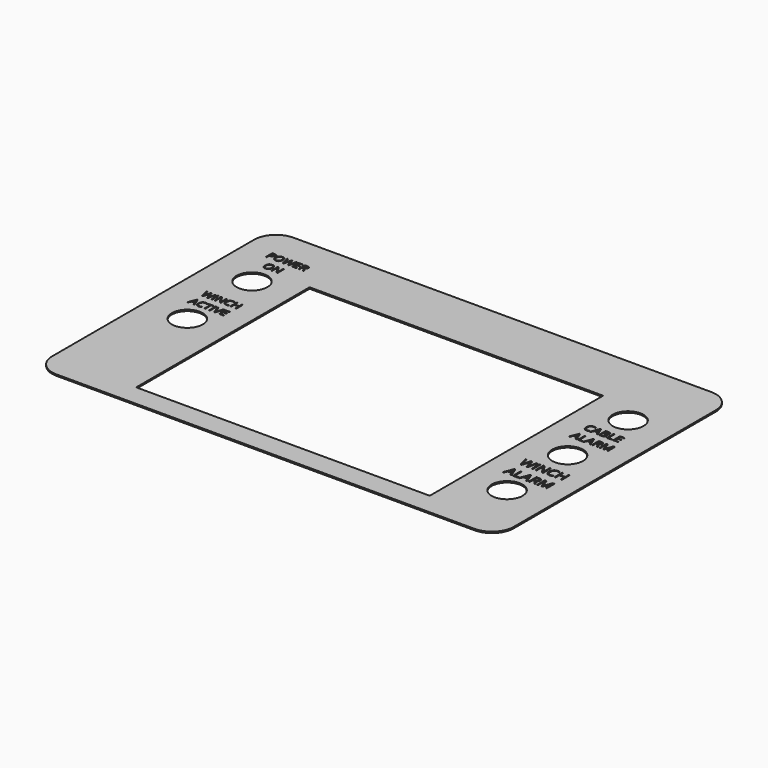
from build123d import *

# Parameters (mm, degrees)
F0_W           = 336.55
F0_H           = 215.9
F0_R           = 11.25
F0_W_2         = 214
F0_H_2         = 158
F1_DEPTH       = 1
F2_R           = 15.88
F3_TEXT_SIZE   = 8.2987464137
F3_TEXT_SIZE_2 = 8.2987425331
F3_TEXT_SIZE_3 = 9.9757634517
F3_TEXT_SIZE_4 = 8.9211467033
F4_DEPTH       = 0.9


# Not quite as in the source:
# - Text() gives the source's letters only with a copy of the font that has no kerning and outlines rounded to 1/6400 em; it was checked with that copy


with BuildPart() as f1:
    # F0 (on Top) → F1 (new body)
    with BuildSketch(Plane.XY):
        Rectangle(F0_W, F0_H)
        with Locations((-137.095, -7.85)):
            Circle(F0_R, mode=Mode.SUBTRACT)
        with Locations((137.095, -59.17)):
            Circle(F0_R, mode=Mode.SUBTRACT)
        with Locations((0, -13.07)):
            Rectangle(F0_W_2, F0_H_2, mode=Mode.SUBTRACT)
        with Locations((137.095, -4.05)):
            Circle(F0_R, mode=Mode.SUBTRACT)
        with Locations((-137.095, 51.07)):
            Circle(F0_R, mode=Mode.SUBTRACT)
        with Locations((137.095, 51.07)):
            Circle(F0_R, mode=Mode.SUBTRACT)
    extrude(amount=F1_DEPTH)

    # F2
    f2_edges = [f1.edges().sort_by_distance(p)[0] for p in [
        (-168.275, -107.95, 0.5),
        (-168.275, 107.95, 0.5),
        (168.275, 107.95, 0.5),
        (168.275, -107.95, 0.5),
    ]]
    fillet(f2_edges, radius=F2_R)

    # F3 (on face) → F4 (cut)
    with BuildSketch(Plane.XY.offset(1)):
        with Locations((-150.6275758147, 79.5598849654)):
            Text('POWER', F3_TEXT_SIZE, font='Open Sans', text_align=(TextAlign.LEFT, TextAlign.BOTTOM))
        with Locations((-144.1584436495, 68.2735898428)):
            Text('ON', F3_TEXT_SIZE, font='Open Sans', text_align=(TextAlign.LEFT, TextAlign.BOTTOM))
        with Locations((-149.8782262206, 19.3607909605)):
            Text('WINCH', F3_TEXT_SIZE_2, font='Open Sans', text_align=(TextAlign.LEFT, TextAlign.BOTTOM))
        with Locations((-149.8782262206, 8.0745011154)):
            Text('ACTIVE', F3_TEXT_SIZE_2, font='Open Sans', text_align=(TextAlign.LEFT, TextAlign.BOTTOM))
        with Locations((121.2788373232, -29.7536514699)):
            Text('WINCH', F3_TEXT_SIZE_3, font='Open Sans', text_align=(TextAlign.LEFT, TextAlign.BOTTOM))
        with Locations((121.2788373232, -43.3206897643)):
            Text('ALARM', F3_TEXT_SIZE_3, font='Open Sans', text_align=(TextAlign.LEFT, TextAlign.BOTTOM))
        with Locations((123.1753826141, 26.5534594655)):
            Text('CABLE', F3_TEXT_SIZE_4, font='Open Sans', text_align=(TextAlign.LEFT, TextAlign.BOTTOM))
        with Locations((123.1753826141, 14.4206999491)):
            Text('ALARM', F3_TEXT_SIZE_4, font='Open Sans', text_align=(TextAlign.LEFT, TextAlign.BOTTOM))
    extrude(amount=-F4_DEPTH, mode=Mode.SUBTRACT)


solid = f1.part
